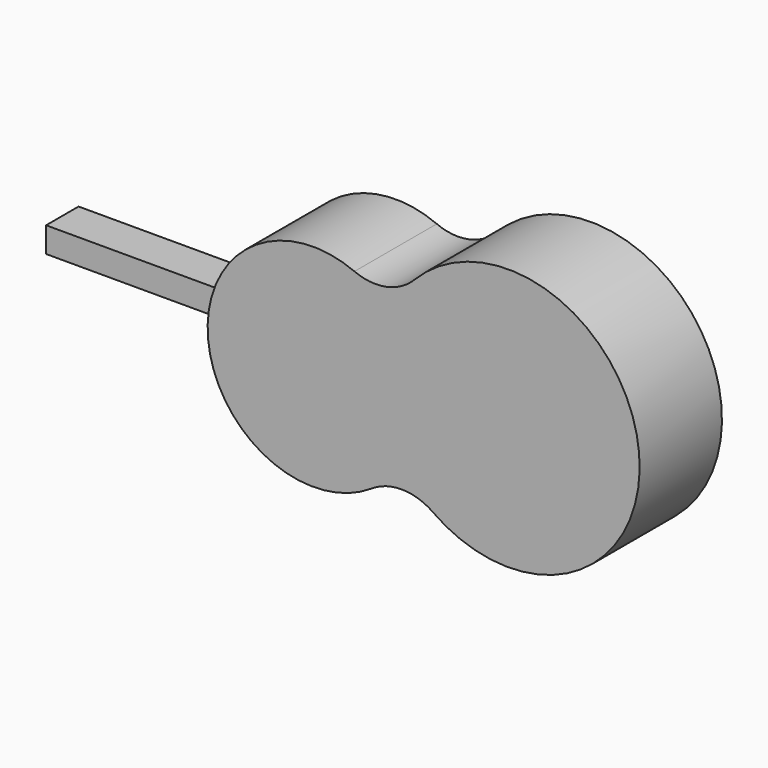
from build123d import *

# Parameters (mm, degrees)
F1_DEPTH = 9.652
F2_W     = 22.6732008159
F2_H     = 1.1748634279
F2_H_2   = 1.2006908655
F3_DEPTH = 3.81
F4_R     = 5.08
F6_DEPTH = 3.556


with BuildPart() as f1:
    # F0 (on Front) → F1 (new body)
    with BuildSketch(Plane.XZ):
        with BuildLine():
            ThreePointArc((-31.5301379097, 29.2723811601), (-9.2584932634, 37.5565839315), (-32.6741015598, 41.6017611729))
            ThreePointArc((-32.6741015598, 41.6017611729), (-49.691111152, 33.8051020972), (-31.5301379097, 29.2723811601))
        make_face()
    extrude(amount=F1_DEPTH)

    # F2 (on Front) → F3 (join)
    with BuildSketch(Plane.XZ):
        with Locations((-58.2245606929, 33.776761964)):
            Rectangle(F2_W, F2_H)
        with Locations((-58.2245606929, 32.5889848173)):
            Rectangle(F2_W, F2_H_2)
    extrude(amount=F3_DEPTH)

    # F4
    f4_edges = [f1.edges().sort_by_distance(p)[0] for p in [
        (-32.674102, -4.826, 41.601761),
        (-31.530138, -4.826, 29.272381),
    ]]
    fillet(f4_edges, radius=F4_R)

    # F5 (on face) → F6 (cut)
    with BuildSketch(Plane(origin=(0, 0, 0), x_dir=(-1, 0, 0), z_dir=(0, 1, 0))):
        with BuildLine():
            ThreePointArc((35.9255568085, 35.9008908942), (32.1931363304, 39.7711420697), (28.1901409202, 36.1814576083))
            Line((28.1901409202, 36.1814576083), (35.9153805385, 35.6203241801))
            ThreePointArc((35.9153805385, 35.6203241801), (35.9230119048, 35.7605152931), (35.9255568085, 35.9008908942))
        make_face()
        with BuildLine():
            Line((35.9153805385, 35.6203241801), (28.1901409202, 36.1814576083))
            ThreePointArc((28.1901409202, 36.1814576083), (31.7721940152, 32.038271085), (35.9153805385, 35.6203241801))
        make_face()
    extrude(amount=-F6_DEPTH, mode=Mode.SUBTRACT)


solid = f1.part
